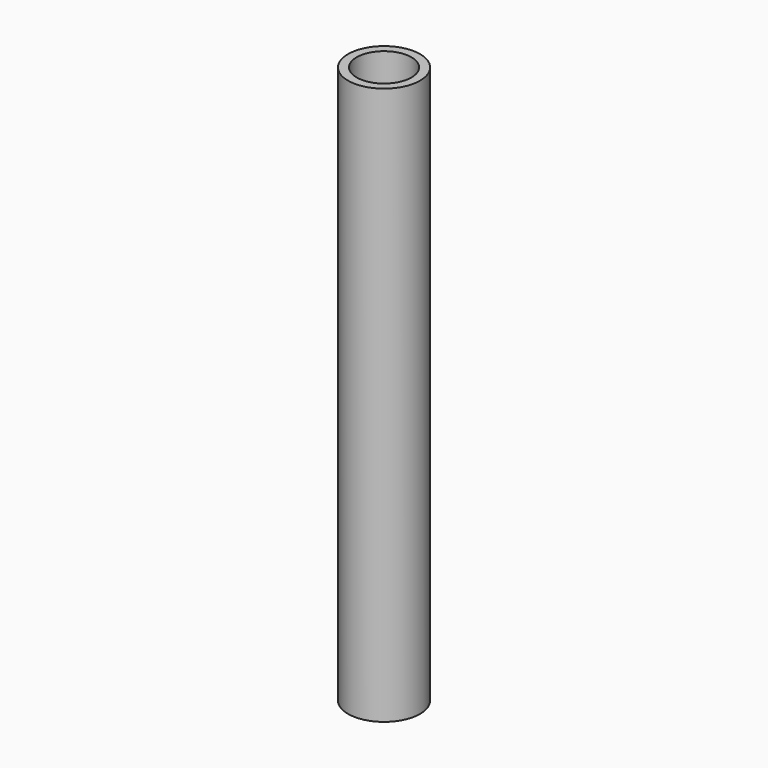
from build123d import *

# Parameters (mm, degrees)
F0_R     = 7.75
F0_R_2   = 5.9
F1_DEPTH = 120


# Not quite as in the source:
# - a feature names something its author has since deleted; it is built from what else it names


with BuildPart() as f1:
    # F0 (on Top) → F1 (new body)
    with BuildSketch(Plane.XY):
        Circle(F0_R)
        Circle(F0_R_2, mode=Mode.SUBTRACT)
    extrude(amount=F1_DEPTH)


solid = f1.part
